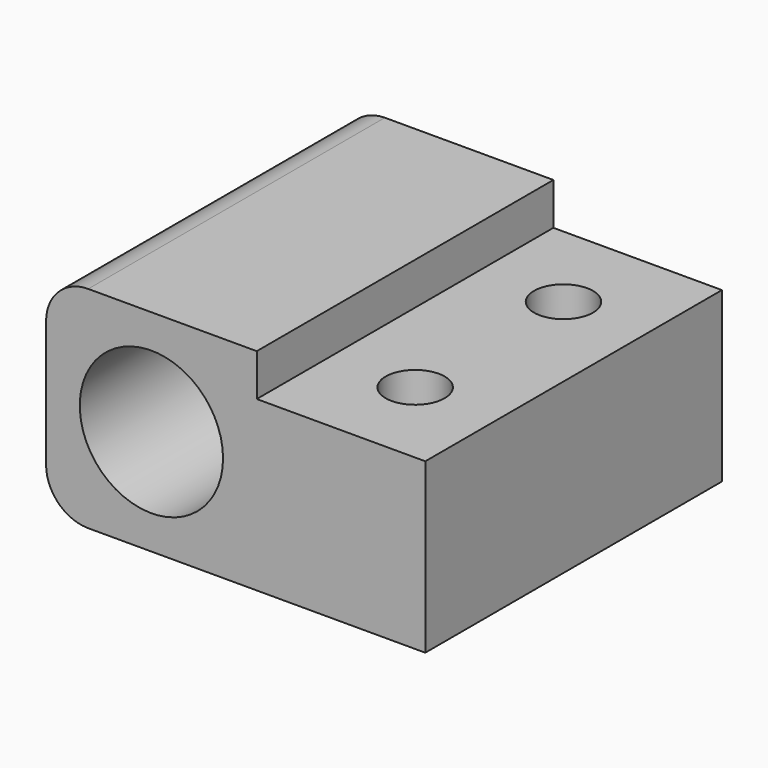
from build123d import *

# Parameters (mm, degrees)
F0_W     = 25
F0_H     = 44
F1_DEPTH = 25
F2_R     = 8.5
F3_DEPTH = 44.001
F0_W_2   = 20
F0_R     = 3.5
F4_DEPTH = 20
F5_R     = 5


# Not quite as in the source:
# - a feature names something its author has since deleted; it is built from what else it names


with BuildPart() as f1:
    # F0 (on Top) → F1 (new body)
    with BuildSketch(Plane.XY):
        Rectangle(F0_W, F0_H)
    extrude(amount=F1_DEPTH)

    # F2 (on face) → F3 (cut, through all)
    with BuildSketch(Plane.XZ.offset(22)):
        with Locations((0, 12.5)):
            Circle(F2_R)
    extrude(amount=-F3_DEPTH, mode=Mode.SUBTRACT)

    # F0 (on Top) → F4 (join)
    with BuildSketch(Plane.XY):
        with Locations((22.5, 0)):
            Rectangle(F0_W_2, F0_H)
        with Locations((22.5, -11)):
            Circle(F0_R, mode=Mode.SUBTRACT)
        with Locations((22.5, 11)):
            Circle(F0_R, mode=Mode.SUBTRACT)
    extrude(amount=F4_DEPTH)

    # F5
    f5_edges = [f1.edges().sort_by_distance(p)[0] for p in [
        (-12.5, 0, 25),
        (-12.5, 0, 0),
    ]]
    fillet(f5_edges, radius=F5_R)


solid = f1.part
